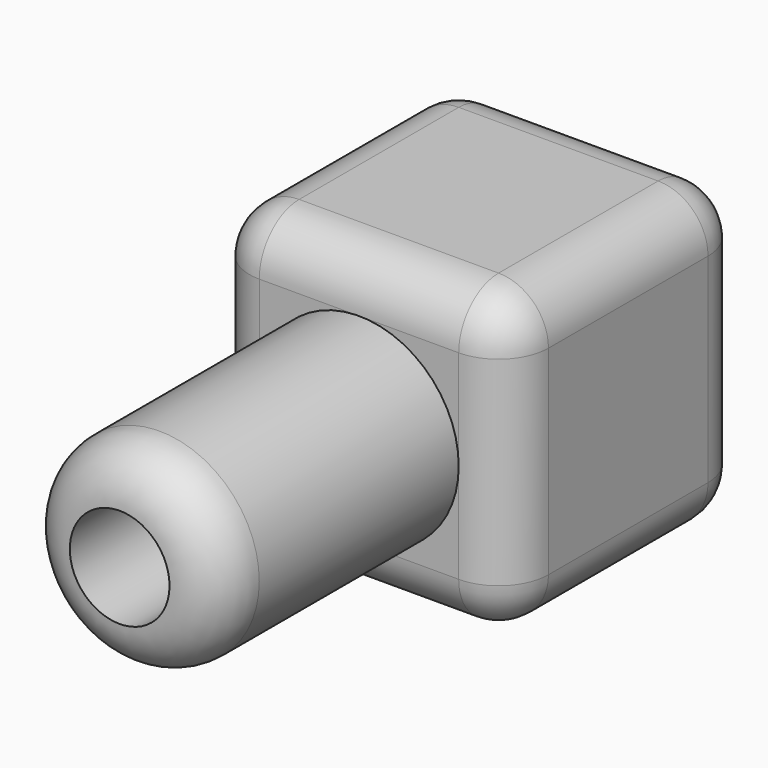
from build123d import *

# Parameters (mm, degrees)
F0_W        = 30
F0_H        = 30
F1_DEPTH    = 30
F2_R        = 10
F3_DEPTH    = 30
F4_R        = 5
F5_DEPTH    = 60.001
F6_R        = 4.99999
F7_T1_DEPTH = 30
F7_T4_ANGLE = 90
F7_T6_ANGLE = 90


# Not quite as in the source:
# - a fillet or chamfer that OpenCascade refuses, or shapes differently, is made with other operations: its cross-section is extruded or revolved along the edge and cut away or added
# - a fillet or chamfer is up to 0.001 mm smaller than in the source, because OpenCascade refuses the exact size


with BuildPart() as f1:
    # F0 (on Front) → F1 (new body)
    with BuildSketch(Plane.XZ):
        Rectangle(F0_W, F0_H)
    extrude(amount=F1_DEPTH)

    # F2 (on face) → F3 (join)
    with BuildSketch(Plane.XZ.offset(30)):
        Circle(F2_R)
    extrude(amount=F3_DEPTH)

    # F4 (on face) → F5 (cut, through all)
    with BuildSketch(Plane.XZ.offset(60)):
        Circle(F4_R)
    extrude(amount=-F5_DEPTH, mode=Mode.SUBTRACT)

    # F6 (radius 5 in the source; OpenCascade refuses exactly that, so slightly less here)
    f6_edges = [f1.edges().sort_by_distance(p)[0] for p in [
        (0, -30, 15),
        (-15, -30, 0),
        (15, -30, 0),
        (0, -30, -15),
        (15, -15, 15),
        (15, -15, -15),
        (15, 0, 0),
        (0, 0, 15),
        (-15, -15, 15),
        (0, 0, -15),
        (-15, 0, 0),
        (-10, -60, 0),
    ]]
    fillet(f6_edges, radius=F6_R)

    # F7: fillet of radius 5 on 2 edges, made by hand

    # F7_s2 → F7_t1 (cut)
    with BuildSketch(Plane.XZ):
        with BuildLine():
            ThreePointArc((-10, -15), (-13.5355339059, -13.5355339059), (-15, -10))
            Line((-15, -10), (-15, -15))
            Line((-15, -15), (-10, -15))
        make_face()
    extrude(amount=F7_T1_DEPTH, mode=Mode.SUBTRACT)

    # F7_s3 → F7_t4 (revolve, cut)
    with BuildSketch(Plane.YZ.offset(-10)):
        with BuildLine():
            ThreePointArc((0, -10.00001), (-1.4644631651, -13.5355368349), (-4.99999, -15))
            Line((-4.99999, -15), (0, -15))
            Line((0, -15), (0, -10.00001))
        make_face()
    revolve(axis=Axis((-10, 0, -10), (0, 1, 0)), revolution_arc=F7_T4_ANGLE, mode=Mode.SUBTRACT)

    # F7_s5 → F7_t6 (revolve, cut)
    with BuildSketch(Plane.XY.offset(-10)):
        with BuildLine():
            ThreePointArc((-10.00001, -30), (-13.5355368349, -28.5355368349), (-15, -25.00001))
            Line((-15, -25.00001), (-15, -30))
            Line((-15, -30), (-10.00001, -30))
        make_face()
    revolve(axis=Axis((-10, -30, -10), (0, -1, 0)), revolution_arc=F7_T6_ANGLE, mode=Mode.SUBTRACT)


solid = f1.part
